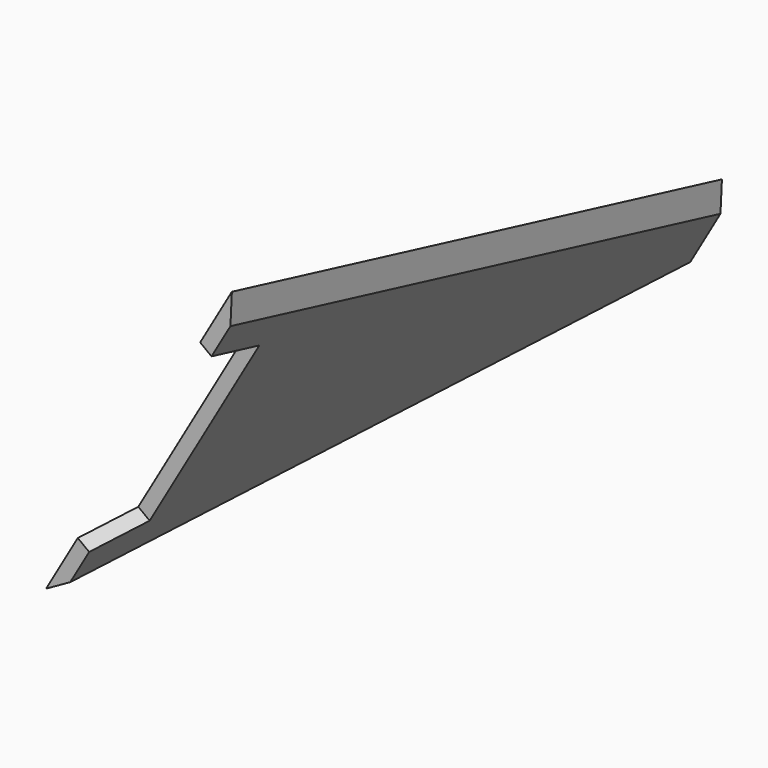
from build123d import *

# Parameters (mm, degrees)
F7_R      = 342.018490112
F8_DEPTH  = 245.8819093468
F10_DEPTH = 134.9414547473
F11_W     = 62.9695011303
F11_H     = 407.8883975744
F12_DEPTH = 201.1136668937
F13_W     = 28.0343884617
F13_H     = 90
F14_DEPTH = 134.9414547473
F17_R     = 326.8037902675
F18_DEPTH = 78.4909831788
F20_R     = 344.6516886149
F21_DEPTH = 6.9809661843


with BuildPart() as f5:
    # F1 (on Front) → F5 section 0
    with BuildSketch(Plane.XZ):
        Polygon((-150, -86.6025403784), (150, -86.6025403784), (0, 173.2050807569), align=None)
    # F4 (on line) → F5 section 1
    with BuildSketch(Plane(origin=(0, 495, 0), x_dir=(-1, 0, 0), z_dir=(0, 1, 0))):
        Polygon((-45, -25.9807621135), (45, -25.9807621135), (0, 51.9615242271), align=None)
    loft()

    # F7 (on face) → F8 (cut, through all)
    with BuildSketch(Plane(origin=(-63.5765006646, 8.9906162556, 36.7059097728), x_dir=(-0.1052740693, -0.9925840823, 0.0607800123), z_dir=(-0.8596030307, 0.1215600245, 0.4962920411))):
        with Locations((-271.4140117168, 0)):
            Circle(F7_R)
    extrude(amount=-F8_DEPTH, mode=Mode.SUBTRACT)

    # F9 (on face) → F10 (cut, through all)
    with BuildSketch(Plane(origin=(-73.8917370326, 10.4493365501, 42.6614142666), x_dir=(-0.1052740693, -0.9925840823, 0.0607800123), z_dir=(-0.8596030307, 0.1215600245, 0.4962920411))):
        Polygon((-39.4725930665, -88.3763476395), (10.5274069335, -98.9037545729), (10.5274069335, 98.9037545729), (-39.4725930665, 88.3763476395), align=None)
    extrude(amount=-F10_DEPTH, mode=Mode.SUBTRACT)

    # F11 (on face) → F12 (cut, through all)
    with BuildSketch(Plane(origin=(-63.5765006646, 8.9906162556, 36.7059097728), x_dir=(0.1052740693, 0.9925840823, -0.0607800123), z_dir=(0.8596030307, -0.1215600245, -0.4962920411))):
        with Locations((-40.5425386316, -31.164906919)):
            Rectangle(F11_W, F11_H)
    extrude(amount=-F12_DEPTH, mode=Mode.SUBTRACT)

    # F13 (on face) → F14 (cut, through all)
    with BuildSketch(Plane(origin=(-73.8917370326, 10.4493365501, 42.6614142666), x_dir=(-0.1052740693, -0.9925840823, 0.0607800123), z_dir=(-0.8596030307, 0.1215600245, 0.4962920411))):
        with Locations((-502.1880928891, 0)):
            Rectangle(F13_W, F13_H)
    extrude(amount=-F14_DEPTH, mode=Mode.SUBTRACT)

    # F17 (on face) → F18 (cut, through all)
    with BuildSketch(Plane(origin=(0, 0, 0), x_dir=(0.8660254038, 0, 0.5), z_dir=(0.5, 0, -0.8660254038))):
        with Locations((-73.8831460476, -254.315674305)):
            Circle(F17_R)
    extrude(amount=F18_DEPTH, mode=Mode.SUBTRACT)

    # F20 (on face) → F21 (cut, through all)
    with BuildSketch(Plane.YZ):
        with Locations((244.284003973, 80.6711390615)):
            Circle(F20_R)
    extrude(amount=F21_DEPTH, mode=Mode.SUBTRACT)


solid = f5.part
